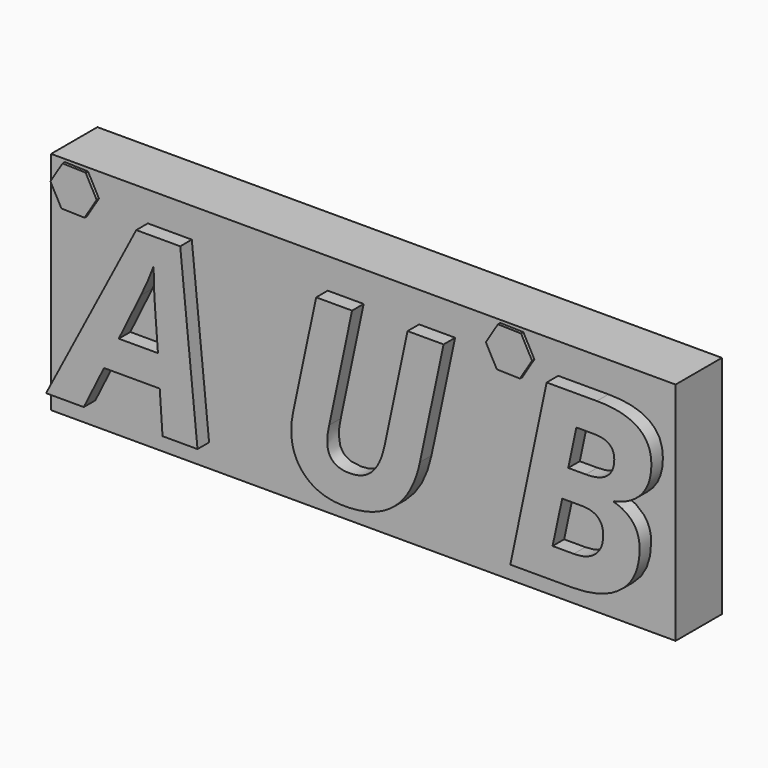
from build123d import *

# Parameters (mm, degrees)
F0_TEXT_SIZE = 52.9166666667
F1_DEPTH     = 9.525
F2_W         = 137.0091959834
F2_H         = 49.5075229555
F3_DEPTH     = 6.35
F5_DEPTH     = 6.985


# Not quite as in the source:
# - Text() gives the source's letters only with a copy of the font that has no kerning and outlines rounded to 1/6400 em; it was checked with that copy


with BuildPart() as f1:
    # F0 (on Front) → F1 (new body, symmetric)
    with BuildSketch(Plane.XZ):
        with Locations((-67.6021054387, -18.8362710178)):
            Text('A U B', F0_TEXT_SIZE, font='Open Sans', font_style=FontStyle.BOLDITALIC, text_align=(TextAlign.LEFT, TextAlign.BOTTOM))
    extrude(amount=F1_DEPTH, both=True)


with BuildPart() as f3:
    # F2 (on Front) → F3 (new body, symmetric)
    with BuildSketch(Plane.XZ):
        with Locations((-3.7126578391, 0.871094875)):
            Rectangle(F2_W, F2_H)
    extrude(amount=F3_DEPTH, both=True)


with BuildPart() as f5:
    # F4 (on Front) → F5 (new body, symmetric)
    with BuildSketch(Plane.XZ):
        Polygon((-64.3754607481, 16.0906464375), (-61.7165611748, 20.4113574377), (-64.1289568766, 24.8743875144), (-69.2002521519, 25.0167065909), (-71.8591517252, 20.6959955908), (-69.4467560234, 16.2329655141), align=None)
    extrude(amount=F5_DEPTH, both=True)


with BuildPart() as f5b:
    # F4 (on Front) → F5, piece 2 (new body, symmetric)
    with BuildSketch(Plane.XZ):
        Polygon((31.1470775296, 16.0906464375), (33.8059771029, 20.4113574377), (31.3935814011, 24.8743875144), (26.3222861258, 25.0167065909), (23.6633865525, 20.6959955908), (26.0757822543, 16.2329655141), align=None)
    extrude(amount=F5_DEPTH, both=True)


solid = Compound([f1.part, f3.part, f5.part, f5b.part])
